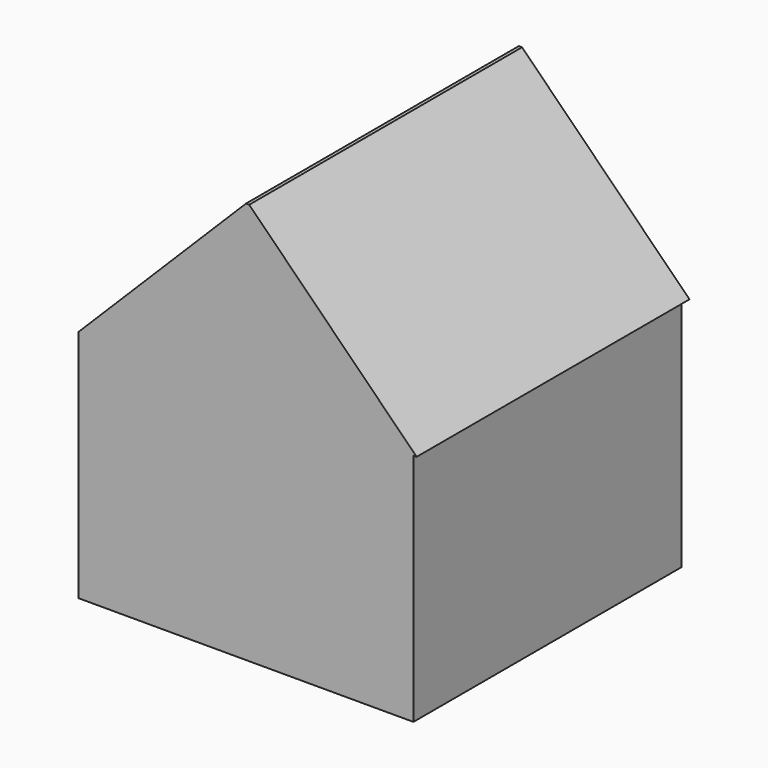
from build123d import *

# Parameters (mm, degrees)
F1_W     = 50.4830703139
F1_H     = 50.9135648608
F2_DEPTH = 25
F0_W     = 50
F0_H     = 50
F0_W_2   = 39.3322317418
F0_H_2   = 39.3322317418
F3_DEPTH = 35
F4_SIZE2 = 24.99999
F4_SIZE  = 24.99999


# Not quite as in the source:
# - a fillet or chamfer is up to 0.001 mm smaller than in the source, because OpenCascade refuses the exact size


with BuildPart() as f2:
    # F1 (on Top) → F2 (new body)
    with BuildSketch(Plane.XY):
        with Locations((25.241535157, 25.4567824304)):
            Rectangle(F1_W, F1_H)
    extrude(amount=F2_DEPTH)

    # F0 (on Top) → F3 (join)
    with BuildSketch(Plane.XY):
        with Locations((25, 25)):
            Rectangle(F0_W, F0_H)
        with Locations((24.6661158709, 24.6661158709)):
            Rectangle(F0_W_2, F0_H_2, mode=Mode.SUBTRACT)
    extrude(amount=-F3_DEPTH)

    # F4 (size 25 and 25 in the source; OpenCascade refuses exactly that, so slightly less here)
    f4_edges = [f2.edges().sort_by_distance(p)[0] for p in [
        (50.48307, 25.456782, 25),
        (0, 25.456782, 25),
    ]]
    chamfer(f4_edges, length=F4_SIZE, length2=F4_SIZE2)


solid = f2.part
